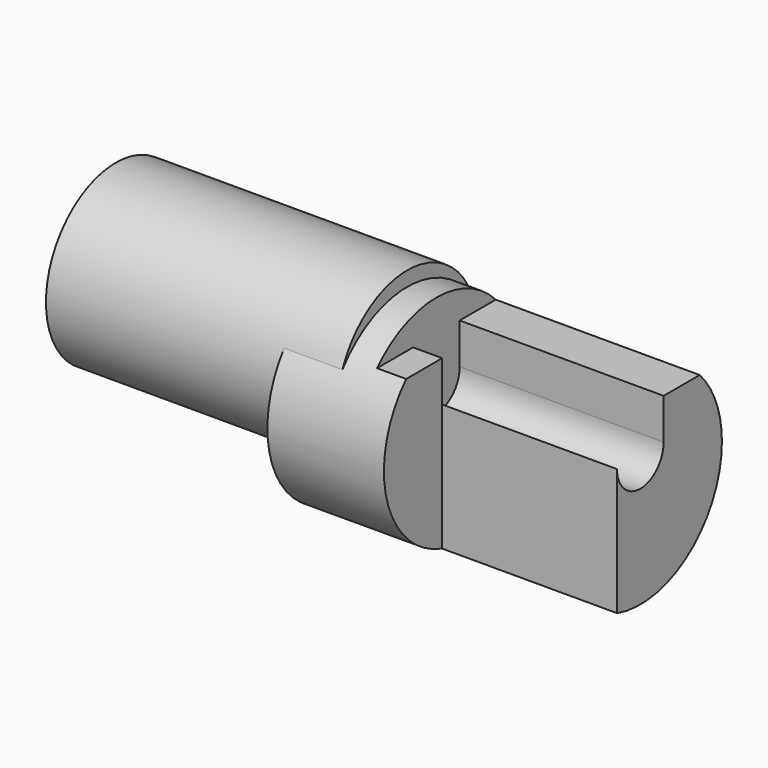
from build123d import *

# Parameters (mm, degrees)
F0_R     = 15
F1_DEPTH = 50
F3_DEPTH = 10
F2_R     = 17.5
F4_DEPTH = 40
F7_DEPTH = 35
F8_DEPTH = 30


with BuildPart() as f1:
    # F0 (on Right) → F1 (new body)
    with BuildSketch(Plane.YZ):
        Circle(F0_R)
    extrude(amount=F1_DEPTH)

    # F2 (on face) → F3 (join)
    with BuildSketch(Plane.YZ.offset(50)):
        with BuildLine():
            ThreePointArc((-13.9053721633, 5.625), (-5.6082968512, -21.5770023354), (17.5, -5))
            ThreePointArc((17.5, -5), (16.5770023354, 0.6082968512), (13.9053721633, 5.625))
            ThreePointArc((13.9053721633, 5.625), (14.7238001625, 2.8652589369), (15, 0))
            ThreePointArc((15, 0), (-2.8652589369, -14.7238001625), (-13.9053721633, 5.625))
        make_face()
        with BuildLine():
            ThreePointArc((15, 0), (14.7238001625, 2.8652589369), (13.9053721633, 5.625))
            ThreePointArc((13.9053721633, 5.625), (0, 12.5), (-13.9053721633, 5.625))
            ThreePointArc((-13.9053721633, 5.625), (-2.8652589369, -14.7238001625), (15, 0))
        make_face()
    extrude(amount=-F3_DEPTH)

    # F2 (on face) → F4 (join)
    with BuildSketch(Plane.YZ.offset(50)):
        with Locations((0, -5)):
            Circle(F2_R)
    extrude(amount=F4_DEPTH)

    # F6 (on face) → F7 (cut)
    with BuildSketch(Plane.YZ.offset(90)):
        with BuildLine():
            ThreePointArc((12.7377392029, 7), (0, 12.5), (-12.7377392029, 7))
            Line((-12.7377392029, 7), (-5, 7))
            Line((-5, 7), (-5, 0))
            ThreePointArc((-5, 0), (0, -5), (5, 0))
            Line((5, 0), (5, 7))
            Line((5, 7), (12.7377392029, 7))
        make_face()
    extrude(amount=-F7_DEPTH, mode=Mode.SUBTRACT)

    # F6 (on face) → F8 (cut)
    with BuildSketch(Plane.YZ.offset(90)):
        with BuildLine():
            Line((-5, 7), (-12.7377392029, 7))
            ThreePointArc((-12.7377392029, 7), (-16.8994794889, -9.5450624864), (-5, -21.7705098312))
            Line((-5, -21.7705098312), (-5, 0))
            Line((-5, 0), (-5, 7))
        make_face()
    extrude(amount=-F8_DEPTH, mode=Mode.SUBTRACT)


solid = f1.part
